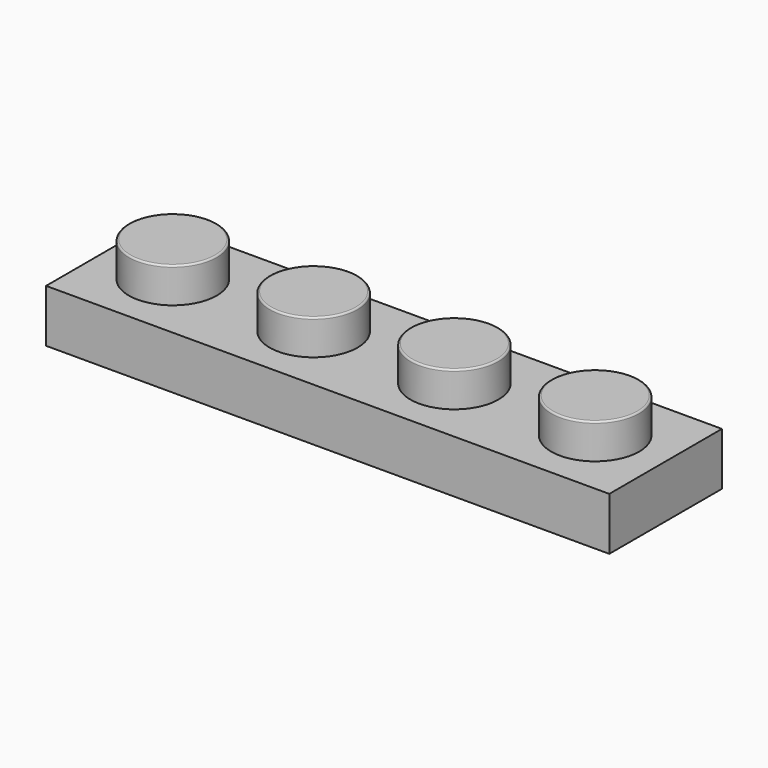
from build123d import *

# Parameters (mm, degrees)
F0_W     = 32
F0_H     = 8
F1_DEPTH = 3
F2_R     = 2.5
F3_DEPTH = 2
F4_R     = 0.1
F5_T     = -1.5
F6_R     = 1.5
F6_R_2   = 0.75
F7_DEPTH = 1.5


# Not quite as in the source:
# - a feature names something its author has since deleted; it is built from what else it names


with BuildPart() as f1:
    # F0 (on Top) → F1 (new body)
    with BuildSketch(Plane.XY):
        Rectangle(F0_W, F0_H)
    extrude(amount=F1_DEPTH)

    # F2 (on face) → F3 (join)
    with BuildSketch(Plane.XY.offset(3)):
        with Locations((-12, 0)):
            Circle(F2_R)
        with Locations((-4, 0)):
            Circle(F2_R)
        with Locations((4, 0)):
            Circle(F2_R)
        with Locations((12, 0)):
            Circle(F2_R)
    extrude(amount=F3_DEPTH)

    # F4
    f4_edges = [f1.edges().sort_by_distance(p)[0] for p in [
        (-14.5, 0, 5),
        (-6.5, 0, 5),
        (1.5, 0, 5),
        (9.5, 0, 5),
    ]]
    fillet(f4_edges, radius=F4_R)

    # F5
    f5_openings = [f1.faces().sort_by_distance(p)[0] for p in [
        (0, 0, 0),
    ]]
    offset(amount=F5_T, openings=f5_openings, kind=Kind.INTERSECTION)

    # F6 (on face) → F7 (join, through all)
    with BuildSketch(Plane(origin=(0, 0, 1.5), x_dir=(1, 0, 0), z_dir=(0, 0, -1))):
        with Locations((-8, 0)):
            Circle(F6_R)
        with Locations((-8, 0)):
            Circle(F6_R_2, mode=Mode.SUBTRACT)
        Circle(F6_R)
        Circle(F6_R_2, mode=Mode.SUBTRACT)
        with Locations((8, 0)):
            Circle(F6_R)
        with Locations((8, 0)):
            Circle(F6_R_2, mode=Mode.SUBTRACT)
    extrude(amount=F7_DEPTH)


solid = f1.part
